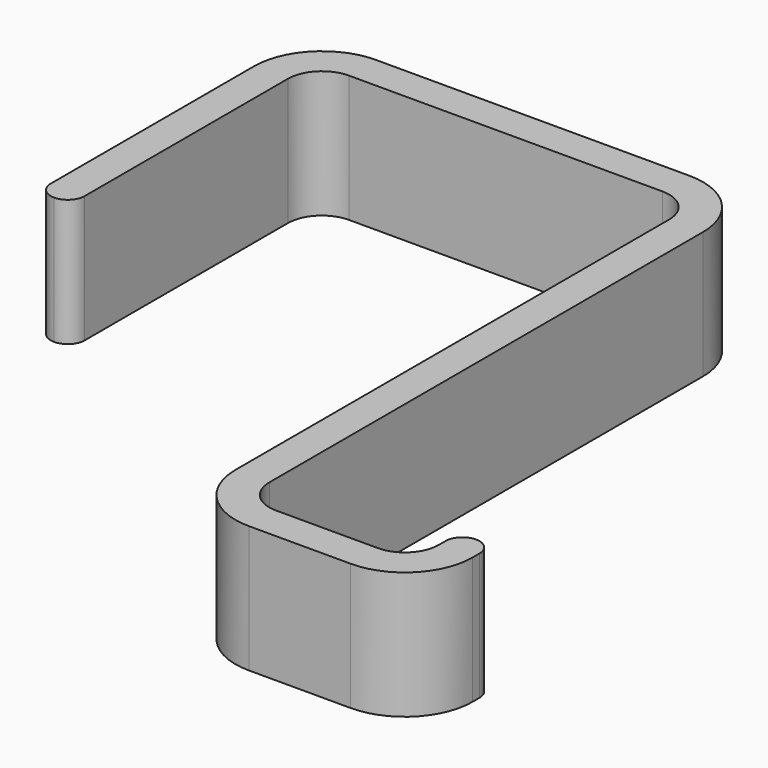
from build123d import *

# Parameters (mm, degrees)
F1_DEPTH = 9.525
F2_R     = 2.54
F3_R     = 5.08
F4_R     = 1.26999


# Not quite as in the source:
# - a fillet or chamfer is up to 0.001 mm smaller than in the source, because OpenCascade refuses the exact size


with BuildPart() as f1:
    # F0 (on Top) → F1 (new body)
    with BuildSketch(Plane.XY):
        Polygon((-28.575, 0), (0, 0), (0, -48.26), (17.78, -48.26), (17.78, -41.275), (15.24, -41.275), (15.24, -45.72), (2.54, -45.72), (2.54, 2.54), (-31.115, 2.54), (-31.115, -22.86), (-28.575, -22.86), align=None)
    extrude(amount=F1_DEPTH)

    # F2
    f2_edges = [f1.edges().sort_by_distance(p)[0] for p in [
        (15.24, -45.72, 4.7625),
        (2.54, -45.72, 4.7625),
        (-28.575, 0, 4.7625),
        (0, 0, 4.7625),
    ]]
    fillet(f2_edges, radius=F2_R)

    # F3
    f3_edges = [f1.edges().sort_by_distance(p)[0] for p in [
        (17.78, -48.26, 4.7625),
        (0, -48.26, 4.7625),
        (2.54, 2.54, 4.7625),
        (-31.115, 2.54, 4.7625),
    ]]
    fillet(f3_edges, radius=F3_R)

    # F4 (radius 1.27 in the source; OpenCascade refuses exactly that, so slightly less here)
    f4_edges = [f1.edges().sort_by_distance(p)[0] for p in [
        (-31.115, -22.86, 4.7625),
        (-28.575, -22.86, 4.7625),
        (15.24, -41.275, 4.7625),
        (17.78, -41.275, 4.7625),
    ]]
    fillet(f4_edges, radius=F4_R)


solid = f1.part
